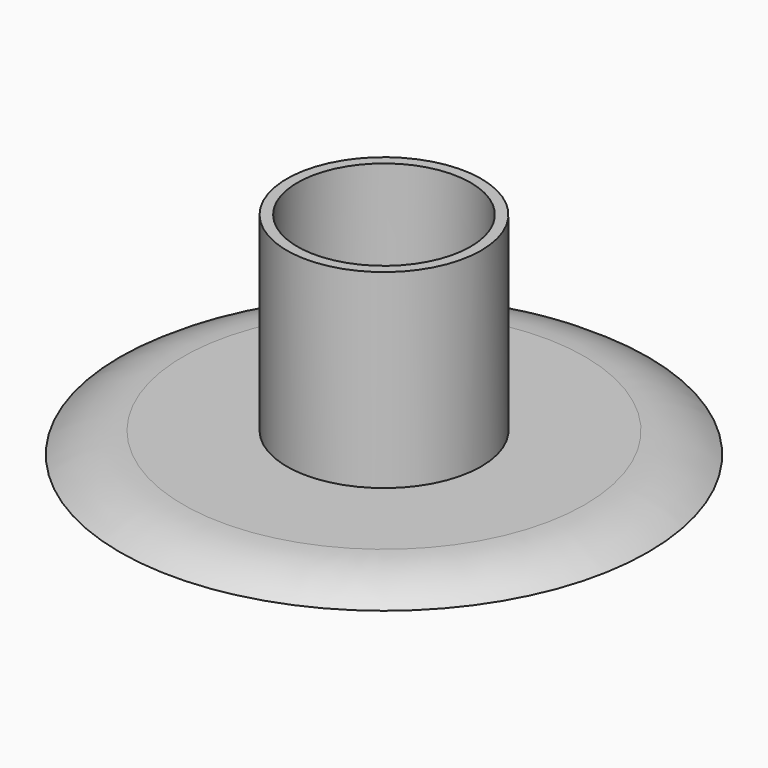
from build123d import *

# Parameters (mm, degrees)
F0_R     = 4.6
F0_R_2   = 4.1
F1_DEPTH = 10
F0_R_3   = 12.5
F2_DEPTH = 1


# Not quite as in the source:
# - a fillet or chamfer that OpenCascade refuses, or shapes differently, is made with other operations: its cross-section is extruded or revolved along the edge and cut away or added


with BuildPart() as f1:
    # F0 (on Top) → F1 (new body)
    with BuildSketch(Plane.XY):
        Circle(F0_R)
        Circle(F0_R_2, mode=Mode.SUBTRACT)
    extrude(amount=F1_DEPTH)


with BuildPart() as f2:
    # F0 (on Top) → F2 (new body)
    with BuildSketch(Plane.XY):
        Circle(F0_R_3)
        Circle(F0_R, mode=Mode.SUBTRACT)
    extrude(amount=F2_DEPTH)

    # F3: fillet of radius 5 on 1 edges, made by hand

    # F3_s1 → F3_t2 (revolve, cut)
    with BuildSketch(Plane.XZ):
        with BuildLine():
            ThreePointArc((12.5, 0), (11.0811388301, 0.7434164903), (9.5, 1))
            Line((9.5, 1), (12.5, 1))
            Line((12.5, 1), (12.5, 0))
        make_face()
    revolve(axis=Axis((0, 0, 1), (0, 0, 1)), mode=Mode.SUBTRACT)


solid = Compound([f1.part, f2.part])
